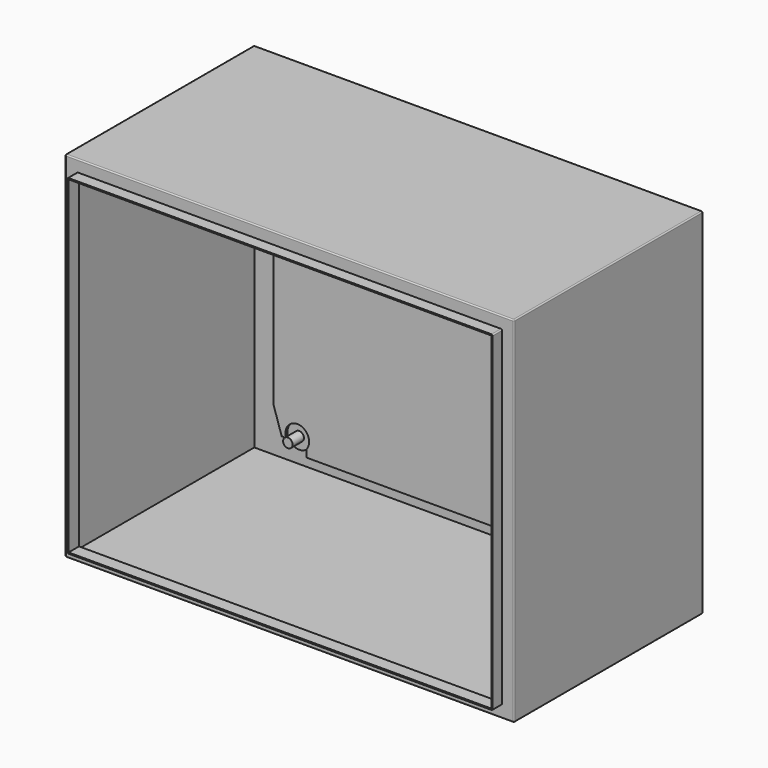
from build123d import *

# Parameters (mm, degrees)
F0_W         = 380
F0_H         = 300
F1_DEPTH     = 200
F2_W         = 360
F2_H         = 280
F3_DEPTH     = 10
F4_R         = 1
F5_T         = 1
F5_T3_DEPTH  = 280
F5_T5_DEPTH  = 360
F5_T8_ANGLE  = 90.000000001
F5_T10_ANGLE = 90.000000001
F5_T12_ANGLE = 90.000000001
F5_T14_ANGLE = 90.000000001
F6_R         = 10
F6_R_2       = 4
F7_DEPTH     = 5
F8_R         = 4
F9_DEPTH     = 12
F11_DEPTH    = 2
F12_R        = 2
F13_DEPTH    = 1.5


# Not quite as in the source:
# - a shell that OpenCascade refuses in one call is made with other operations: the cavity is built on its own and cut out


with BuildPart() as f1:
    # F0 (on Front) → F1 (new body)
    with BuildSketch(Plane.XZ):
        Rectangle(F0_W, F0_H)
    extrude(amount=F1_DEPTH)

    # F2 (on face) → F3 (join)
    with BuildSketch(Plane.XZ.offset(200)):
        Rectangle(F2_W, F2_H)
    extrude(amount=F3_DEPTH)

    # F4
    f4_edges = [f1.edges().sort_by_distance(p)[0] for p in [
        (190, -100, 150),
        (190, -200, 0),
        (190, -100, -150),
        (190, 0, 0),
        (0, -200, 150),
        (-190, -100, 150),
        (-190, -100, -150),
        (-190, -200, 0),
        (-190, 0, 0),
        (0, 0, 150),
        (0, -200, -150),
        (0, 0, -150),
        (180, -205, 140),
        (-180, -205, 140),
        (180, -205, -140),
        (-180, -205, -140),
    ]]
    fillet(f4_edges, radius=F4_R)

    # F5: shell of thickness 1, made by hand


with BuildPart() as f5_core1:
    # F5_t2: copy of F1
    add(f1.part)

    # the walls: a layer under each face that stays
    f5_faces = [f5_core1.faces().sort_by_distance(p)[0] for p in [
        (190, -100, 0),
        (0, -100, 150),
        (0, 0, 0),
        (129.9375, -200, -145.3209876543),
        (0, -100, -150),
        (180, -205, 0),
        (0, -205, -140),
        (0, -205, 140),
        (-180, -205, 0),
        (-190, -100, 0),
    ]]
    thicken(f5_faces, amount=-F5_T, mode=Mode.SUBTRACT)

    # F5_s4 → F5_t3 (cut)
    with BuildSketch(Plane.XY.offset(-140)):
        Polygon((180.01, -200.01), (180, -199), (179, -199), (179, -200), align=None)
        Polygon((-180.01, -200.01), (-180, -199), (-179, -199), (-179, -200), align=None)
    extrude(amount=F5_T3_DEPTH, mode=Mode.SUBTRACT)

    # F5_s6 → F5_t5 (cut)
    with BuildSketch(Plane.YZ.offset(-180)):
        Polygon((-200.01, -140.01), (-199, -140), (-199, -139), (-200, -139), align=None)
        Polygon((-200.01, 140.01), (-199, 140), (-199, 139), (-200, 139), align=None)
    extrude(amount=F5_T5_DEPTH, mode=Mode.SUBTRACT)

    # F5_s7 → F5_t8 (revolve, cut)
    with BuildSketch(Plane.XY.offset(-139)):
        Polygon((180.01, -200.01), (180, -199), (179, -199), (179, -200), align=None)
    revolve(axis=Axis((179, -200, -139), (0, 1, 0)), revolution_arc=F5_T8_ANGLE, mode=Mode.SUBTRACT)

    # F5_s9 → F5_t10 (revolve, cut)
    with BuildSketch(Plane.XY.offset(139)):
        Polygon((180.01, -200.01), (180, -199), (179, -199), (179, -200), align=None)
    revolve(axis=Axis((179, -200, 139), (0, -1, 0)), revolution_arc=F5_T10_ANGLE, mode=Mode.SUBTRACT)

    # F5_s11 → F5_t12 (revolve, cut)
    with BuildSketch(Plane.XY.offset(-139)):
        Polygon((-180.01, -200.01), (-180, -199), (-179, -199), (-179, -200), align=None)
    revolve(axis=Axis((-179, -200, -139), (0, -1, 0)), revolution_arc=F5_T12_ANGLE, mode=Mode.SUBTRACT)

    # F5_s13 → F5_t14 (revolve, cut)
    with BuildSketch(Plane.YZ.offset(-179)):
        Polygon((-200.01, 140.01), (-199, 140), (-199, 139), (-200, 139), align=None)
    revolve(axis=Axis((-179, -200, 139), (0, -1, 0)), revolution_arc=F5_T14_ANGLE, mode=Mode.SUBTRACT)


with BuildPart() as f1_1:
    add(f1.part)

    # what is left inside the walls is the cavity
    f5_cavity = [f5_core1.part.solids().sort_by_distance(p)[0] for p in [
        (0, -1.01, -49.666667),
    ]]
    add(f5_cavity, mode=Mode.SUBTRACT)

    # F6 (on face) → F7 (join)
    with BuildSketch(Plane.XZ.offset(1)):
        with Locations((-147, -125)):
            Circle(F6_R)
        with Locations((-147, -125)):
            Circle(F6_R_2, mode=Mode.SUBTRACT)
        with Locations((-147, -125)):
            Circle(F6_R_2)
        with Locations((147, 125)):
            Circle(F6_R)
        with Locations((147, 125)):
            Circle(F6_R_2, mode=Mode.SUBTRACT)
        with Locations((147, 125)):
            Circle(F6_R_2)
        with Locations((-147, 125)):
            Circle(F6_R)
        with Locations((-147, 125)):
            Circle(F6_R_2, mode=Mode.SUBTRACT)
        with Locations((-147, 125)):
            Circle(F6_R_2)
        with Locations((147, -125)):
            Circle(F6_R)
        with Locations((147, -125)):
            Circle(F6_R_2, mode=Mode.SUBTRACT)
        with Locations((147, -125)):
            Circle(F6_R_2)
    extrude(amount=F7_DEPTH)

    # F8 (on face) → F9 (join)
    with BuildSketch(Plane.XZ.offset(6)):
        with Locations((-147, 125)):
            Circle(F8_R)
        with Locations((147, 125)):
            Circle(F8_R)
        with Locations((-147, -125)):
            Circle(F8_R)
        with Locations((147, -125)):
            Circle(F8_R)
    extrude(amount=F9_DEPTH)


with BuildPart() as f11:
    # F10 (on face) → F11 (new body)
    with BuildSketch(Plane.XZ.offset(6)):
        with BuildLine():
            Line((139, 125), (139, 137.5))
            Line((139, 137.5), (-139, 137.5))
            Line((-139, 137.5), (-139, 125))
            ThreePointArc((-139, 125), (-148.7958315233, 117.2041684767), (-154.193747285, 128.5))
            Line((-154.193747285, 128.5), (-160.193747285, 128.5))
            Line((-160.193747285, 128.5), (-167, 107.5))
            Line((-167, 107.5), (-167, -107.5))
            Line((-167, -107.5), (-160.1938831182, -128.4995809004))
            Line((-160.1938831182, -128.4995809004), (-156.3676202463, -128.4996701162))
            ThreePointArc((-156.3676202463, -128.4996701162), (-148.7781728737, -115.1593647953), (-137, -125))
            ThreePointArc((-137, -125), (-137.5131670195, -128.1622776602), (-139, -131))
            Line((-139, -131), (-139, -137.5))
            Line((-139, -137.5), (-137, -137.5))
            Line((-137, -137.5), (139, -137.5))
            Line((139, -137.5), (139, -125))
            ThreePointArc((139, -125), (148.7958315233, -117.2041684767), (154.193747285, -128.5))
            Line((154.193747285, -128.5), (160.193747285, -128.5))
            Line((160.193747285, -128.5), (167, -107.5))
            Line((167, -107.5), (167, 107.5))
            Line((167, 107.5), (160.193747285, 128.5))
            Line((160.193747285, 128.5), (154.193747285, 128.5))
            ThreePointArc((154.193747285, 128.5), (148.7958315233, 117.2041684767), (139, 125))
        make_face()
    extrude(amount=F11_DEPTH)

    # F12 (on face) → F13 (join)
    with BuildSketch(Plane.XZ.offset(8)):
        with Locations((52, 2.5)):
            Circle(F12_R)
    extrude(amount=F13_DEPTH)


solid = Compound([f1_1.part, f11.part])
